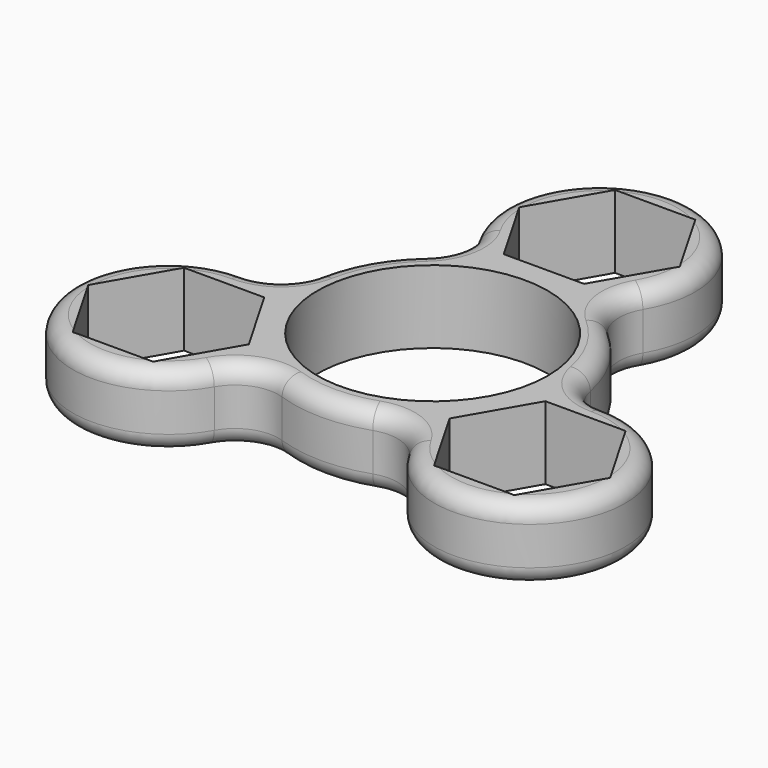
from build123d import *

# Parameters (mm, degrees)
F0_R         = 13.25
F1_DEPTH     = 8.4
F2_T2_ANGLE  = 241.2097411279
F2_T4_ANGLE  = 241.2097411279
F2_T6_ANGLE  = 38.0438050379
F2_T8_ANGLE  = 38.0438050379
F2_T10_ANGLE = 79.6267730829
F2_T12_ANGLE = 79.6267730829
F2_T14_ANGLE = 241.2097411279
F2_T16_ANGLE = 241.2097411279
F2_T18_ANGLE = 79.6267730829
F2_T20_ANGLE = 79.6267730829
F2_T22_ANGLE = 38.0438050379
F2_T24_ANGLE = 38.0438050379
F2_T26_ANGLE = 79.6267730829
F2_T28_ANGLE = 79.6267730829
F2_T30_ANGLE = 241.2097411279
F2_T32_ANGLE = 241.2097411279
F2_T34_ANGLE = 79.6267730829
F2_T36_ANGLE = 79.6267730829
F2_T38_ANGLE = 38.0438050379
F2_T40_ANGLE = 38.0438050379
F2_T42_ANGLE = 79.6267730829
F2_T44_ANGLE = 79.6267730829
F2_T46_ANGLE = 79.6267730829
F2_T48_ANGLE = 79.6267730829


# Not quite as in the source:
# - a fillet or chamfer that OpenCascade refuses, or shapes differently, is made with other operations: its cross-section is extruded or revolved along the edge and cut away or added


with BuildPart() as f1:
    # F0 (on Top) → F1 (new body)
    with BuildSketch(Plane.XY):
        with BuildLine():
            ThreePointArc((-11.2007987683, -17.3991266146), (-8.6193611443, -15.1788828445), (-5.2148732009, -15.1263048197))
            ThreePointArc((-5.2148732009, -15.1263048197), (0, -16), (5.2148732009, -15.1263048197))
            ThreePointArc((5.2148732009, -15.1263048197), (8.6193611443, -15.1788828445), (11.2007987683, -17.3991266146))
            ThreePointArc((11.2007987683, -17.3991266146), (30.3108891325, -17.5), (20.6684850361, -1.0006129687))
            ThreePointArc((20.6684850361, -1.0006129687), (17.4549787165, 0.1248557069), (15.7072008397, 3.0469397403))
            ThreePointArc((15.7072008397, 3.0469397403), (13.8564064606, 8), (10.4923276388, 12.0793650794))
            ThreePointArc((10.4923276388, 12.0793650794), (8.8356175722, 15.0540271376), (9.4676862678, 18.3997395833))
            ThreePointArc((9.4676862678, 18.3997395833), (0, 35), (-9.4676862678, 18.3997395833))
            ThreePointArc((-9.4676862678, 18.3997395833), (-8.8356175722, 15.0540271376), (-10.4923276388, 12.0793650794))
            ThreePointArc((-10.4923276388, 12.0793650794), (-13.8564064606, 8), (-15.7072008397, 3.0469397403))
            ThreePointArc((-15.7072008397, 3.0469397403), (-17.4549787165, 0.1248557069), (-20.6684850361, -1.0006129687))
            ThreePointArc((-20.6684850361, -1.0006129687), (-30.3108891325, -17.5), (-11.2007987683, -17.3991266146))
        make_face()
        Polygon((-16.1658075373, -20), (-25.4034118443, -20), (-30.0222139979, -12), (-25.4034118443, -4), (-16.1658075373, -4), (-11.5470053838, -12), align=None, mode=Mode.SUBTRACT)
        Polygon((25.4034118443, -4), (30.0222139979, -12), (25.4034118443, -20), (16.1658075373, -20), (11.5470053838, -12), (16.1658075373, -4), align=None, mode=Mode.SUBTRACT)
        Circle(F0_R, mode=Mode.SUBTRACT)
        Polygon((9.237604307, 24), (4.6188021535, 16), (-4.6188021535, 16), (-9.237604307, 24), (-4.6188021535, 32), (4.6188021535, 32), align=None, mode=Mode.SUBTRACT)
    extrude(amount=F1_DEPTH)

    # F2: fillet of radius 2 on 24 edges, made by hand

    # F2_s1 → F2_t2 (revolve, cut)
    with BuildSketch(Plane(origin=(10.5166628713, 17.7792561849, 0), x_dir=(0, 0, 1), z_dir=(-0.5091145833, -0.8606987516, 0))):
        with BuildLine():
            ThreePointArc((6.4, 1.21875), (7.8142135624, 1.8045364376), (8.4, 3.21875))
            Line((8.4, 3.21875), (8.4, 1.21875))
            Line((8.4, 1.21875), (6.4, 1.21875))
        make_face()
    revolve(axis=Axis((0, 24, 8.4), (0, 0, 1)), revolution_arc=F2_T2_ANGLE, mode=Mode.SUBTRACT)

    # F2_s3 → F2_t4 (revolve, cut)
    with BuildSketch(Plane(origin=(10.5166628713, 17.7792561849, 0), x_dir=(0, 0, 1), z_dir=(-0.5091145833, -0.8606987516, 0))):
        with BuildLine():
            ThreePointArc((2, 1.21875), (0.5857864376, 1.8045364376), (0, 3.21875))
            Line((0, 3.21875), (0, 1.21875))
            Line((0, 1.21875), (2, 1.21875))
        make_face()
    revolve(axis=Axis((0, 24, 0), (0, 0, 1)), revolution_arc=F2_T4_ANGLE, mode=Mode.SUBTRACT)

    # F2_s5 → F2_t6 (revolve, cut)
    with BuildSketch(Plane(origin=(0, 0, 0), x_dir=(0, 0, 1), z_dir=(0.7549603175, 0.6557704774, 0))):
        with BuildLine():
            ThreePointArc((2, -16), (0.5857864376, -15.4142135624), (0, -14))
            Line((0, -14), (0, -16))
            Line((0, -16), (2, -16))
        make_face()
    revolve(axis=Axis((0, 0, 0), (0, 0, 1)), revolution_arc=F2_T6_ANGLE, mode=Mode.SUBTRACT)

    # F2_s7 → F2_t8 (revolve, cut)
    with BuildSketch(Plane(origin=(0, 0, 0), x_dir=(0, 0, 1), z_dir=(0.7549603175, 0.6557704774, 0))):
        with BuildLine():
            ThreePointArc((6.4, -16), (7.8142135624, -15.4142135624), (8.4, -14))
            Line((8.4, -14), (8.4, -16))
            Line((8.4, -16), (6.4, -16))
        make_face()
    revolve(axis=Axis((0, 0, 8.4), (0, 0, 1)), revolution_arc=F2_T8_ANGLE, mode=Mode.SUBTRACT)

    # F2_s9 → F2_t10 (revolve, cut)
    with BuildSketch(Plane(origin=(0, 0, 0), x_dir=(0, 0, 1), z_dir=(0.1904337338, 0.9817000525, 0))):
        with BuildLine():
            ThreePointArc((2, -16), (0.5857864376, -15.4142135624), (0, -14))
            Line((0, -14), (0, -16))
            Line((0, -16), (2, -16))
        make_face()
    revolve(axis=Axis((-20.6157011021, 3.9991084092, 0), (0, 0, -1)), revolution_arc=F2_T10_ANGLE, mode=Mode.SUBTRACT)

    # F2_s11 → F2_t12 (revolve, cut)
    with BuildSketch(Plane(origin=(0, 0, 0), x_dir=(0, 0, 1), z_dir=(0.1904337338, 0.9817000525, 0))):
        with BuildLine():
            ThreePointArc((6.4, -16), (7.8142135624, -15.4142135624), (8.4, -14))
            Line((8.4, -14), (8.4, -16))
            Line((8.4, -16), (6.4, -16))
        make_face()
    revolve(axis=Axis((-20.6157011021, 3.9991084092, 8.4), (0, 0, -1)), revolution_arc=F2_T12_ANGLE, mode=Mode.SUBTRACT)

    # F2_s13 → F2_t14 (revolve, cut)
    with BuildSketch(Plane(origin=(-20.6556189522, 0.2180691172, 0), x_dir=(0, 0, 1), z_dir=(0.9999442756, -0.0105567868, 0))):
        with BuildLine():
            ThreePointArc((2, 1.21875), (0.5857864376, 1.8045364376), (0, 3.21875))
            Line((0, 3.21875), (0, 1.21875))
            Line((0, 1.21875), (2, 1.21875))
        make_face()
    revolve(axis=Axis((-20.7846096908, -12, 0), (0, 0, 1)), revolution_arc=F2_T14_ANGLE, mode=Mode.SUBTRACT)

    # F2_s15 → F2_t16 (revolve, cut)
    with BuildSketch(Plane(origin=(-20.6556189522, 0.2180691172, 0), x_dir=(0, 0, 1), z_dir=(0.9999442756, -0.0105567868, 0))):
        with BuildLine():
            ThreePointArc((6.4, 1.21875), (7.8142135624, 1.8045364376), (8.4, 3.21875))
            Line((8.4, 3.21875), (8.4, 1.21875))
            Line((8.4, 1.21875), (6.4, 1.21875))
        make_face()
    revolve(axis=Axis((-20.7846096908, -12, 8.4), (0, 0, 1)), revolution_arc=F2_T16_ANGLE, mode=Mode.SUBTRACT)

    # F2_s17 → F2_t18 (revolve, cut)
    with BuildSketch(Plane(origin=(-10.1389560808, -17.9973253021, 0), x_dir=(0, 0, 1), z_dir=(-0.4908296922, -0.8712555384, 0))):
        with BuildLine():
            ThreePointArc((2, 1.21875), (0.5857864376, 1.8045364376), (0, 3.21875))
            Line((0, 3.21875), (0, 1.21875))
            Line((0, 1.21875), (2, 1.21875))
        make_face()
    revolve(axis=Axis((-6.8445210762, -19.8532750758, 0), (0, 0, -1)), revolution_arc=F2_T18_ANGLE, mode=Mode.SUBTRACT)

    # F2_s19 → F2_t20 (revolve, cut)
    with BuildSketch(Plane(origin=(-10.1389560808, -17.9973253021, 0), x_dir=(0, 0, 1), z_dir=(-0.4908296922, -0.8712555384, 0))):
        with BuildLine():
            ThreePointArc((6.4, 1.21875), (7.8142135624, 1.8045364376), (8.4, 3.21875))
            Line((8.4, 3.21875), (8.4, 1.21875))
            Line((8.4, 1.21875), (6.4, 1.21875))
        make_face()
    revolve(axis=Axis((-6.8445210762, -19.8532750758, 8.4), (0, 0, -1)), revolution_arc=F2_T20_ANGLE, mode=Mode.SUBTRACT)

    # F2_s21 → F2_t22 (revolve, cut)
    with BuildSketch(Plane(origin=(0, 0, 0), x_dir=(0, 0, 1), z_dir=(-0.9453940512, 0.3259295751, 0))):
        with BuildLine():
            ThreePointArc((2, -16), (0.5857864376, -15.4142135624), (0, -14))
            Line((0, -14), (0, -16))
            Line((0, -16), (2, -16))
        make_face()
    revolve(axis=Axis((0, 0, 0), (0, 0, 1)), revolution_arc=F2_T22_ANGLE, mode=Mode.SUBTRACT)

    # F2_s23 → F2_t24 (revolve, cut)
    with BuildSketch(Plane(origin=(0, 0, 0), x_dir=(0, 0, 1), z_dir=(-0.9453940512, 0.3259295751, 0))):
        with BuildLine():
            ThreePointArc((6.4, -16), (7.8142135624, -15.4142135624), (8.4, -14))
            Line((8.4, -14), (8.4, -16))
            Line((8.4, -16), (6.4, -16))
        make_face()
    revolve(axis=Axis((0, 0, 8.4), (0, 0, 1)), revolution_arc=F2_T24_ANGLE, mode=Mode.SUBTRACT)

    # F2_s25 → F2_t26 (revolve, cut)
    with BuildSketch(Plane(origin=(0, 0, 0), x_dir=(0, 0, 1), z_dir=(-0.9453940512, -0.3259295751, 0))):
        with BuildLine():
            ThreePointArc((2, -16), (0.5857864376, -15.4142135624), (0, -14))
            Line((0, -14), (0, -16))
            Line((0, -16), (2, -16))
        make_face()
    revolve(axis=Axis((6.8445210762, -19.8532750758, 0), (0, 0, -1)), revolution_arc=F2_T26_ANGLE, mode=Mode.SUBTRACT)

    # F2_s27 → F2_t28 (revolve, cut)
    with BuildSketch(Plane(origin=(0, 0, 0), x_dir=(0, 0, 1), z_dir=(-0.9453940512, -0.3259295751, 0))):
        with BuildLine():
            ThreePointArc((6.4, -16), (7.8142135624, -15.4142135624), (8.4, -14))
            Line((8.4, -14), (8.4, -16))
            Line((8.4, -16), (6.4, -16))
        make_face()
    revolve(axis=Axis((6.8445210762, -19.8532750758, 8.4), (0, 0, -1)), revolution_arc=F2_T28_ANGLE, mode=Mode.SUBTRACT)

    # F2_s29 → F2_t30 (revolve, cut)
    with BuildSketch(Plane(origin=(10.1389560808, -17.9973253021, 0), x_dir=(0, 0, 1), z_dir=(-0.4908296922, 0.8712555384, 0))):
        with BuildLine():
            ThreePointArc((2, 1.21875), (0.5857864376, 1.8045364376), (0, 3.21875))
            Line((0, 3.21875), (0, 1.21875))
            Line((0, 1.21875), (2, 1.21875))
        make_face()
    revolve(axis=Axis((20.7846096908, -12, 0), (0, 0, 1)), revolution_arc=F2_T30_ANGLE, mode=Mode.SUBTRACT)

    # F2_s31 → F2_t32 (revolve, cut)
    with BuildSketch(Plane(origin=(10.1389560808, -17.9973253021, 0), x_dir=(0, 0, 1), z_dir=(-0.4908296922, 0.8712555384, 0))):
        with BuildLine():
            ThreePointArc((6.4, 1.21875), (7.8142135624, 1.8045364376), (8.4, 3.21875))
            Line((8.4, 3.21875), (8.4, 1.21875))
            Line((8.4, 1.21875), (6.4, 1.21875))
        make_face()
    revolve(axis=Axis((20.7846096908, -12, 8.4), (0, 0, 1)), revolution_arc=F2_T32_ANGLE, mode=Mode.SUBTRACT)

    # F2_s33 → F2_t34 (revolve, cut)
    with BuildSketch(Plane(origin=(20.6556189522, 0.2180691172, 0), x_dir=(0, 0, 1), z_dir=(0.9999442756, 0.0105567868, 0))):
        with BuildLine():
            ThreePointArc((2, 1.21875), (0.5857864376, 1.8045364376), (0, 3.21875))
            Line((0, 3.21875), (0, 1.21875))
            Line((0, 1.21875), (2, 1.21875))
        make_face()
    revolve(axis=Axis((20.6157011021, 3.9991084092, 0), (0, 0, -1)), revolution_arc=F2_T34_ANGLE, mode=Mode.SUBTRACT)

    # F2_s35 → F2_t36 (revolve, cut)
    with BuildSketch(Plane(origin=(20.6556189522, 0.2180691172, 0), x_dir=(0, 0, 1), z_dir=(0.9999442756, 0.0105567868, 0))):
        with BuildLine():
            ThreePointArc((6.4, 1.21875), (7.8142135624, 1.8045364376), (8.4, 3.21875))
            Line((8.4, 3.21875), (8.4, 1.21875))
            Line((8.4, 1.21875), (6.4, 1.21875))
        make_face()
    revolve(axis=Axis((20.6157011021, 3.9991084092, 8.4), (0, 0, -1)), revolution_arc=F2_T36_ANGLE, mode=Mode.SUBTRACT)

    # F2_s37 → F2_t38 (revolve, cut)
    with BuildSketch(Plane(origin=(0, 0, 0), x_dir=(0, 0, 1), z_dir=(0.1904337338, -0.9817000525, 0))):
        with BuildLine():
            ThreePointArc((2, -16), (0.5857864376, -15.4142135624), (0, -14))
            Line((0, -14), (0, -16))
            Line((0, -16), (2, -16))
        make_face()
    revolve(axis=Axis((0, 0, 0), (0, 0, 1)), revolution_arc=F2_T38_ANGLE, mode=Mode.SUBTRACT)

    # F2_s39 → F2_t40 (revolve, cut)
    with BuildSketch(Plane(origin=(0, 0, 0), x_dir=(0, 0, 1), z_dir=(0.1904337338, -0.9817000525, 0))):
        with BuildLine():
            ThreePointArc((6.4, -16), (7.8142135624, -15.4142135624), (8.4, -14))
            Line((8.4, -14), (8.4, -16))
            Line((8.4, -16), (6.4, -16))
        make_face()
    revolve(axis=Axis((0, 0, 8.4), (0, 0, 1)), revolution_arc=F2_T40_ANGLE, mode=Mode.SUBTRACT)

    # F2_s41 → F2_t42 (revolve, cut)
    with BuildSketch(Plane(origin=(0, 0, 0), x_dir=(0, 0, 1), z_dir=(0.7549603175, -0.6557704774, 0))):
        with BuildLine():
            ThreePointArc((2, -16), (0.5857864376, -15.4142135624), (0, -14))
            Line((0, -14), (0, -16))
            Line((0, -16), (2, -16))
        make_face()
    revolve(axis=Axis((13.7711800259, 15.8541666667, 0), (0, 0, -1)), revolution_arc=F2_T42_ANGLE, mode=Mode.SUBTRACT)

    # F2_s43 → F2_t44 (revolve, cut)
    with BuildSketch(Plane(origin=(0, 0, 0), x_dir=(0, 0, 1), z_dir=(0.7549603175, -0.6557704774, 0))):
        with BuildLine():
            ThreePointArc((6.4, -16), (7.8142135624, -15.4142135624), (8.4, -14))
            Line((8.4, -14), (8.4, -16))
            Line((8.4, -16), (6.4, -16))
        make_face()
    revolve(axis=Axis((13.7711800259, 15.8541666667, 8.4), (0, 0, -1)), revolution_arc=F2_T44_ANGLE, mode=Mode.SUBTRACT)

    # F2_s45 → F2_t46 (revolve, cut)
    with BuildSketch(Plane(origin=(-10.5166628713, 17.7792561849, 0), x_dir=(0, 0, 1), z_dir=(-0.5091145833, 0.8606987516, 0))):
        with BuildLine():
            ThreePointArc((2, 1.21875), (0.5857864376, 1.8045364376), (0, 3.21875))
            Line((0, 3.21875), (0, 1.21875))
            Line((0, 1.21875), (2, 1.21875))
        make_face()
    revolve(axis=Axis((-13.7711800259, 15.8541666667, 0), (0, 0, -1)), revolution_arc=F2_T46_ANGLE, mode=Mode.SUBTRACT)

    # F2_s47 → F2_t48 (revolve, cut)
    with BuildSketch(Plane(origin=(-10.5166628713, 17.7792561849, 0), x_dir=(0, 0, 1), z_dir=(-0.5091145833, 0.8606987516, 0))):
        with BuildLine():
            ThreePointArc((6.4, 1.21875), (7.8142135624, 1.8045364376), (8.4, 3.21875))
            Line((8.4, 3.21875), (8.4, 1.21875))
            Line((8.4, 1.21875), (6.4, 1.21875))
        make_face()
    revolve(axis=Axis((-13.7711800259, 15.8541666667, 8.4), (0, 0, -1)), revolution_arc=F2_T48_ANGLE, mode=Mode.SUBTRACT)


solid = f1.part
